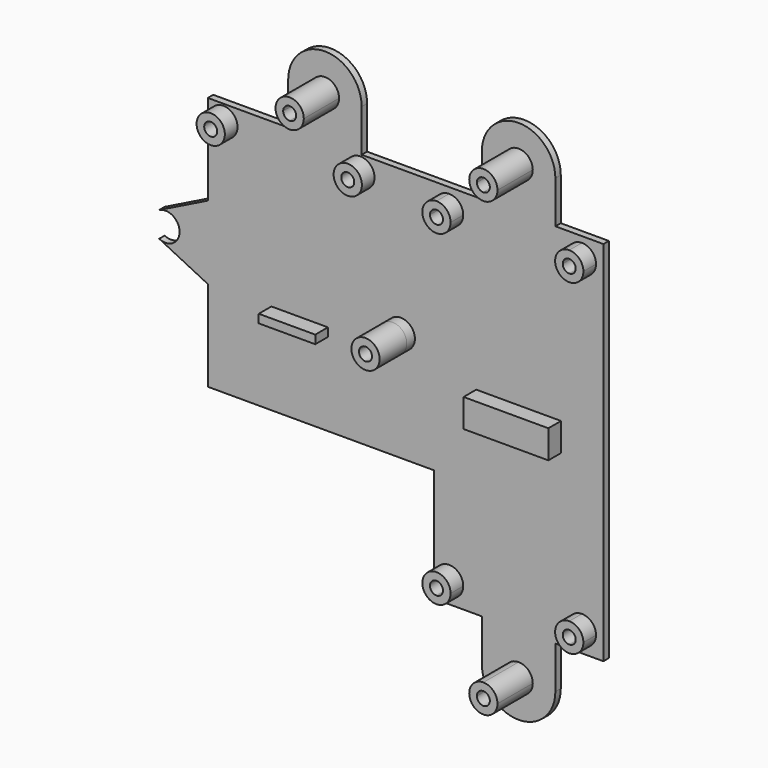
from build123d import *

# Parameters (mm, degrees)
F1_DEPTH = 4
F0_R     = 2.5
F2_DEPTH = 1.2
F3_DEPTH = 9
F0_R_2   = 1.15
F4_DEPTH = 3


# Not quite as in the source:
# - a feature names something its author has since deleted; it is built from what else it names


with BuildPart() as f1:
    # F0 (on Front) → F1 (new body)
    with BuildSketch(Plane.XZ):
        with BuildLine():
            ThreePointArc((-51.5757481032, 29.6725835079), (-54.0757481032, 32.1725835079), (-56.5757481032, 29.6725835079))
            ThreePointArc((-56.5757481032, 29.6725835079), (-54.0757481032, 27.1725835079), (-51.5757481032, 29.6725835079))
        make_face()
        with BuildLine():
            ThreePointArc((-52.9257481032, 29.6725835079), (-54.0757481032, 28.5225835079), (-55.2257481032, 29.6725835079))
            ThreePointArc((-55.2257481032, 29.6725835079), (-54.0757481032, 30.8225835079), (-52.9257481032, 29.6725835079))
        make_face(mode=Mode.SUBTRACT)
    extrude(amount=F1_DEPTH)


with BuildPart() as f1b:
    # F0 (on Front) → F1, piece 2 (new body)
    with BuildSketch(Plane.XZ):
        with BuildLine():
            Line((-28.6757481032, 29.6725835079), (-27.3257481032, 29.6725835079))
            ThreePointArc((-27.3257481032, 29.6725835079), (-29.8257481032, 32.1725835079), (-32.3257481032, 29.6725835079))
            Line((-32.3257481032, 29.6725835079), (-30.9757481032, 29.6725835079))
            ThreePointArc((-30.9757481032, 29.6725835079), (-29.8257481032, 30.8225835079), (-28.6757481032, 29.6725835079))
        make_face()
        with BuildLine():
            ThreePointArc((-32.3257481032, 29.6725835079), (-29.8257481032, 27.1725835079), (-27.3257481032, 29.6725835079))
            Line((-27.3257481032, 29.6725835079), (-28.6757481032, 29.6725835079))
            ThreePointArc((-28.6757481032, 29.6725835079), (-29.8257481032, 28.5225835079), (-30.9757481032, 29.6725835079))
            Line((-30.9757481032, 29.6725835079), (-32.3257481032, 29.6725835079))
        make_face()
    extrude(amount=F1_DEPTH)


with BuildPart() as f1c:
    # F0 (on Front) → F1, piece 3 (new body)
    with BuildSketch(Plane.XZ):
        with BuildLine():
            ThreePointArc((-11.6263987731, 28.95), (-12.3586318202, 30.717766953), (-14.1263987731, 31.45))
            Line((-14.1263987731, 31.45), (-14.1263987731, 30.1))
            ThreePointArc((-14.1263987731, 30.1), (-13.3132259748, 29.7631727984), (-12.9763987731, 28.95))
            Line((-12.9763987731, 28.95), (-11.6263987731, 28.95))
        make_face()
        with BuildLine():
            Line((-14.1263987731, 30.1), (-14.1263987731, 31.45))
            ThreePointArc((-14.1263987731, 31.45), (-15.8941657261, 30.717766953), (-16.6263987731, 28.95))
            Line((-16.6263987731, 28.95), (-15.2763987731, 28.95))
            ThreePointArc((-15.2763987731, 28.95), (-14.9395715715, 29.7631727984), (-14.1263987731, 30.1))
        make_face()
        with BuildLine():
            Line((-15.2763987731, 28.95), (-16.6263987731, 28.95))
            ThreePointArc((-16.6263987731, 28.95), (-16.4189081118, 27.9528034637), (-15.8308780274, 27.1211341023))
            ThreePointArc((-15.8308780274, 27.1211341023), (-13.1292022368, 26.6574906613), (-11.6263987731, 28.95))
            Line((-11.6263987731, 28.95), (-12.9763987731, 28.95))
            ThreePointArc((-12.9763987731, 28.95), (-14.1263987731, 27.8), (-15.2763987731, 28.95))
        make_face()
    extrude(amount=F1_DEPTH)


with BuildPart() as f1d:
    # F0 (on Front) → F1, piece 4 (new body)
    with BuildSketch(Plane.XZ):
        with BuildLine():
            ThreePointArc((9.3736012269, 31.45), (7.6058342739, 30.717766953), (6.8736012269, 28.95))
            Line((6.8736012269, 28.95), (8.2236012269, 28.95))
            ThreePointArc((8.2236012269, 28.95), (8.5604284285, 29.7631727984), (9.3736012269, 30.1))
            Line((9.3736012269, 30.1), (9.3736012269, 31.45))
        make_face()
        with BuildLine():
            Line((8.2236012269, 28.95), (6.8736012269, 28.95))
            ThreePointArc((6.8736012269, 28.95), (7.6058342739, 27.182233047), (9.3736012269, 26.45))
            Line((9.3736012269, 26.45), (9.3736012269, 27.8))
            ThreePointArc((9.3736012269, 27.8), (8.5604284285, 28.1368272016), (8.2236012269, 28.95))
        make_face()
        with BuildLine():
            ThreePointArc((11.8736012269, 28.95), (11.1413681798, 30.717766953), (9.3736012269, 31.45))
            Line((9.3736012269, 31.45), (9.3736012269, 30.1))
            ThreePointArc((9.3736012269, 30.1), (10.1867740252, 29.7631727984), (10.5236012269, 28.95))
            ThreePointArc((10.5236012269, 28.95), (10.1867740252, 28.1368272016), (9.3736012269, 27.8))
            Line((9.3736012269, 27.8), (9.3736012269, 26.45))
            ThreePointArc((9.3736012269, 26.45), (11.1413681798, 27.182233047), (11.8736012269, 28.95))
        make_face()
    extrude(amount=F1_DEPTH)


with BuildPart() as f1e:
    # F0 (on Front) → F1, piece 5 (new body)
    with BuildSketch(Plane.XZ):
        with BuildLine():
            ThreePointArc((-11.6263987731, -28.85), (-15.8941657261, -27.082233047), (-14.1263987731, -31.35))
            ThreePointArc((-14.1263987731, -31.35), (-12.3586318202, -30.617766953), (-11.6263987731, -28.85))
        make_face()
        with BuildLine():
            ThreePointArc((-12.9763987731, -28.85), (-13.3132259748, -29.6631727984), (-14.1263987731, -30))
            ThreePointArc((-14.1263987731, -30), (-14.9395715715, -28.0368272016), (-12.9763987731, -28.85))
        make_face(mode=Mode.SUBTRACT)
    extrude(amount=F1_DEPTH)


with BuildPart() as f1f:
    # F0 (on Front) → F1, piece 6 (new body)
    with BuildSketch(Plane.XZ):
        with BuildLine():
            ThreePointArc((11.8736012269, -28.85), (11.1413681798, -27.082233047), (9.3736012269, -26.35))
            ThreePointArc((9.3736012269, -26.35), (6.8736012269, -28.85), (9.3736012269, -31.35))
            ThreePointArc((9.3736012269, -31.35), (11.1413681798, -30.617766953), (11.8736012269, -28.85))
        make_face()
        with BuildLine():
            ThreePointArc((10.5236012269, -28.85), (10.1867740252, -29.6631727984), (9.3736012269, -30))
            ThreePointArc((9.3736012269, -30), (8.5604284285, -28.0368272016), (10.5236012269, -28.85))
        make_face(mode=Mode.SUBTRACT)
    extrude(amount=F1_DEPTH)


with BuildPart() as f1g:
    # F0 (on Front) → F1, piece 7 (new body)
    with BuildSketch(Plane.XZ):
        Polygon((-35.5757481032, 3.6725835079), (-40.5757481032, 3.6725835079), (-45.5757481032, 3.6725835079), (-45.5757481032, 2.1725835079), (-35.5757481032, 2.1725835079), align=None)
    extrude(amount=F1_DEPTH)


with BuildPart() as f1h:
    # F0 (on Front) → F1, piece 8 (new body)
    with BuildSketch(Plane.XZ):
        Polygon((5.6736012269, 2.5), (-1.8263987731, 2.5), (-9.3263987731, 2.5), (-9.3263987731, -2.5), (5.6736012269, -2.5), align=None)
    extrude(amount=F1_DEPTH)


with BuildPart() as f2:
    # F0 (on Front) → F2 (new body)
    with BuildSketch(Plane.XZ):
        with BuildLine():
            Line((-14.1263987731, 32.5), (-16.8263987731, 32.5))
            Line((-16.8263987731, 32.5), (-16.8263987731, 28.95))
            Line((-16.8263987731, 28.95), (-16.6263987731, 28.95))
            ThreePointArc((-16.6263987731, 28.95), (-15.8941657261, 30.717766953), (-14.1263987731, 31.45))
            Line((-14.1263987731, 31.45), (-14.1263987731, 32.5))
        make_face()
        with BuildLine():
            Line((-16.8263987731, 28.95), (-16.8263987731, 32.5))
            Line((-16.8263987731, 32.5), (-29.6046157777, 32.5))
            Line((-29.6046157777, 32.5), (-36.1046157777, 32.5))
            Line((-36.1046157777, 32.5), (-42.6046157777, 32.5))
            Line((-42.6046157777, 32.5), (-56.8263987731, 32.5))
            Line((-56.8263987731, 32.5), (-56.8263987731, 29.6725835079))
            Line((-56.8263987731, 29.6725835079), (-56.5757481032, 29.6725835079))
            ThreePointArc((-56.5757481032, 29.6725835079), (-54.0757481032, 32.1725835079), (-51.5757481032, 29.6725835079))
            Line((-51.5757481032, 29.6725835079), (-51.3257481032, 29.6725835079))
            Line((-51.3257481032, 29.6725835079), (-40.5757481032, 29.6725835079))
            Line((-40.5757481032, 29.6725835079), (-32.3257481032, 29.6725835079))
            ThreePointArc((-32.3257481032, 29.6725835079), (-29.8257481032, 32.1725835079), (-27.3257481032, 29.6725835079))
            Line((-27.3257481032, 29.6725835079), (-27.3257481032, 20.5483327715))
            Line((-27.3257481032, 20.5483327715), (-16.8263987731, 20.68381793))
            Line((-16.8263987731, 20.68381793), (-16.8263987731, 27.1211341023))
            Line((-16.8263987731, 27.1211341023), (-16.8263987731, 28.95))
        make_face()
        with BuildLine():
            Line((-8.3263987731, 32.5), (-14.1263987731, 32.5))
            Line((-14.1263987731, 32.5), (-14.1263987731, 31.45))
            ThreePointArc((-14.1263987731, 31.45), (-12.3586318202, 30.717766953), (-11.6263987731, 28.95))
            Line((-11.6263987731, 28.95), (-1.8263987731, 28.95))
            Line((-1.8263987731, 28.95), (-1.8263987731, 32.5))
            Line((-1.8263987731, 32.5), (-8.3263987731, 32.5))
        make_face()
        with BuildLine():
            Line((-16.6263987731, 28.95), (-16.8263987731, 28.95))
            Line((-16.8263987731, 28.95), (-16.8263987731, 27.1211341023))
            Line((-16.8263987731, 27.1211341023), (-15.8308780274, 27.1211341023))
            ThreePointArc((-15.8308780274, 27.1211341023), (-16.4189081118, 27.9528034637), (-16.6263987731, 28.95))
        make_face()
        with BuildLine():
            Line((-36.1046157777, 32.5), (-29.6046157777, 32.5))
            Line((-29.6046157777, 32.5), (-29.6046157777, 40))
            ThreePointArc((-29.6046157777, 40), (-31.5084217, 35.4038059223), (-36.1046157777, 33.5))
            Line((-36.1046157777, 33.5), (-36.1046157777, 32.5))
        make_face()
        with BuildLine():
            Line((-8.3263987731, 40), (-8.3263987731, 32.5))
            Line((-8.3263987731, 32.5), (-1.8263987731, 32.5))
            Line((-1.8263987731, 32.5), (-1.8263987731, 33.5))
            ThreePointArc((-1.8263987731, 33.5), (-6.4225928508, 35.4038059223), (-8.3263987731, 40))
        make_face()
        with BuildLine():
            Line((-15.8308780274, 27.1211341023), (-16.8263987731, 27.1211341023))
            Line((-16.8263987731, 27.1211341023), (-16.8263987731, 20.68381793))
            Line((-16.8263987731, 20.68381793), (-16.8263987731, 10))
            Line((-16.8263987731, 10), (-1.8263987731, 10))
            Line((-1.8263987731, 10), (-1.8263987731, 28.95))
            Line((-1.8263987731, 28.95), (-11.6263987731, 28.95))
            ThreePointArc((-11.6263987731, 28.95), (-13.1292022368, 26.6574906613), (-15.8308780274, 27.1211341023))
        make_face()
        with BuildLine():
            Line((-42.6046157777, 32.5), (-36.1046157777, 32.5))
            Line((-36.1046157777, 32.5), (-36.1046157777, 33.5))
            ThreePointArc((-36.1046157777, 33.5), (-40.7008098554, 35.4038059223), (-42.6046157777, 40))
            Line((-42.6046157777, 40), (-42.6046157777, 32.5))
        make_face()
        with BuildLine():
            Line((-33.6046157777, 40), (-29.6046157777, 40))
            ThreePointArc((-29.6046157777, 40), (-36.1046157777, 46.5), (-42.6046157777, 40))
            Line((-42.6046157777, 40), (-38.6046157777, 40))
            ThreePointArc((-38.6046157777, 40), (-36.1046157777, 42.5), (-33.6046157777, 40))
        make_face()
        with BuildLine():
            ThreePointArc((-36.1046157777, 33.5), (-31.5084217, 35.4038059223), (-29.6046157777, 40))
            Line((-29.6046157777, 40), (-33.6046157777, 40))
            ThreePointArc((-33.6046157777, 40), (-34.3368488248, 38.232233047), (-36.1046157777, 37.5))
            Line((-36.1046157777, 37.5), (-36.1046157777, 33.5))
        make_face()
        with BuildLine():
            Line((-1.8263987731, 33.5), (-1.8263987731, 32.5))
            Line((-1.8263987731, 32.5), (4.6736012269, 32.5))
            Line((4.6736012269, 32.5), (4.6736012269, 40))
            ThreePointArc((4.6736012269, 40), (2.7697953046, 35.4038059223), (-1.8263987731, 33.5))
        make_face()
        with BuildLine():
            Line((4.6736012269, 32.5), (-1.8263987731, 32.5))
            Line((-1.8263987731, 32.5), (-1.8263987731, 28.95))
            Line((-1.8263987731, 28.95), (6.8736012269, 28.95))
            ThreePointArc((6.8736012269, 28.95), (7.6058342739, 30.717766953), (9.3736012269, 31.45))
            Line((9.3736012269, 31.45), (9.3736012269, 32.5))
            Line((9.3736012269, 32.5), (4.6736012269, 32.5))
        make_face()
        with BuildLine():
            Line((-4.3263987731, 40), (-8.3263987731, 40))
            ThreePointArc((-8.3263987731, 40), (-6.4225928508, 35.4038059223), (-1.8263987731, 33.5))
            Line((-1.8263987731, 33.5), (-1.8263987731, 37.5))
            ThreePointArc((-1.8263987731, 37.5), (-3.5941657261, 38.232233047), (-4.3263987731, 40))
        make_face()
        with BuildLine():
            ThreePointArc((4.6736012269, 40), (-1.8263987731, 46.5), (-8.3263987731, 40))
            Line((-8.3263987731, 40), (-4.3263987731, 40))
            ThreePointArc((-4.3263987731, 40), (-1.8263987731, 42.5), (0.6736012269, 40))
            Line((0.6736012269, 40), (4.6736012269, 40))
        make_face()
        Polygon((-16.8263987731, 10), (-16.8263987731, 20.68381793), (-27.3257481032, 20.5483327715), (-27.3257481032, 10), align=None)
        with BuildLine():
            ThreePointArc((-42.6046157777, 40), (-40.7008098554, 35.4038059223), (-36.1046157777, 33.5))
            Line((-36.1046157777, 33.5), (-36.1046157777, 37.5))
            ThreePointArc((-36.1046157777, 37.5), (-37.8723827307, 38.232233047), (-38.6046157777, 40))
            Line((-38.6046157777, 40), (-42.6046157777, 40))
        make_face()
        with BuildLine():
            Line((6.8736012269, 28.95), (-1.8263987731, 28.95))
            Line((-1.8263987731, 28.95), (-1.8263987731, 10))
            Line((-1.8263987731, 10), (9.3736012269, 10))
            Line((9.3736012269, 10), (9.3736012269, 26.45))
            ThreePointArc((9.3736012269, 26.45), (7.6058342739, 27.182233047), (6.8736012269, 28.95))
        make_face()
        with BuildLine():
            Line((-1.8263987731, 37.5), (-1.8263987731, 33.5))
            ThreePointArc((-1.8263987731, 33.5), (2.7697953046, 35.4038059223), (4.6736012269, 40))
            Line((4.6736012269, 40), (0.6736012269, 40))
            ThreePointArc((0.6736012269, 40), (-0.0586318202, 38.232233047), (-1.8263987731, 37.5))
        make_face()
        with BuildLine():
            Line((-1.8263987731, 10), (-16.8263987731, 10))
            Line((-16.8263987731, 10), (-16.8263987731, -12.5))
            Line((-16.8263987731, -12.5), (-16.8263987731, -32.5))
            Line((-16.8263987731, -32.5), (-14.1263987731, -32.5))
            Line((-14.1263987731, -32.5), (-8.3263987731, -32.5))
            Line((-8.3263987731, -32.5), (-1.8263987731, -32.5))
            Line((-1.8263987731, -32.5), (4.6736012269, -32.5))
            Line((4.6736012269, -32.5), (9.3736012269, -32.5))
            Line((9.3736012269, -32.5), (9.3736012269, -31.35))
            ThreePointArc((9.3736012269, -31.35), (6.8736012269, -28.85), (9.3736012269, -26.35))
            Line((9.3736012269, -26.35), (9.3736012269, 10))
            Line((9.3736012269, 10), (-1.8263987731, 10))
        make_face()
        with BuildLine():
            ThreePointArc((-11.6263987731, -28.85), (-12.3586318202, -30.617766953), (-14.1263987731, -31.35))
            ThreePointArc((-14.1263987731, -31.35), (-15.8941657261, -27.082233047), (-11.6263987731, -28.85))
        make_face(mode=Mode.SUBTRACT)
        Polygon((-9.3263987731, 2.5), (-1.8263987731, 2.5), (5.6736012269, 2.5), (5.6736012269, -2.5), (-9.3263987731, -2.5), align=None, mode=Mode.SUBTRACT)
        Polygon((-16.8263987731, -12.5), (-16.8263987731, 10), (-27.3257481032, 10), (-40.5757481032, 10), (-56.8263987731, 10), (-56.8263987731, 3.5), (-56.8263987731, -12.5), align=None)
        Polygon((-45.5757481032, 3.6725835079), (-40.5757481032, 3.6725835079), (-35.5757481032, 3.6725835079), (-35.5757481032, 2.1725835079), (-45.5757481032, 2.1725835079), align=None, mode=Mode.SUBTRACT)
        with Locations((-22.6864659105, 6.8783217843)):
            Circle(F0_R, mode=Mode.SUBTRACT)
        with BuildLine():
            Line((-27.3257481032, 10), (-27.3257481032, 20.5483327715))
            Line((-27.3257481032, 20.5483327715), (-27.3257481032, 29.6725835079))
            ThreePointArc((-27.3257481032, 29.6725835079), (-29.8257481032, 27.1725835079), (-32.3257481032, 29.6725835079))
            Line((-32.3257481032, 29.6725835079), (-40.5757481032, 29.6725835079))
            Line((-40.5757481032, 29.6725835079), (-40.5757481032, 10))
            Line((-40.5757481032, 10), (-27.3257481032, 10))
        make_face()
        with BuildLine():
            Line((13.1736012269, 32.5), (9.3736012269, 32.5))
            Line((9.3736012269, 32.5), (9.3736012269, 31.45))
            ThreePointArc((9.3736012269, 31.45), (11.1413681798, 30.717766953), (11.8736012269, 28.95))
            ThreePointArc((11.8736012269, 28.95), (11.1413681798, 27.182233047), (9.3736012269, 26.45))
            Line((9.3736012269, 26.45), (9.3736012269, 10))
            Line((9.3736012269, 10), (13.1736012269, 10))
            Line((13.1736012269, 10), (13.1736012269, 32.5))
        make_face()
        with BuildLine():
            Line((-56.5757481032, 29.6725835079), (-56.8263987731, 29.6725835079))
            Line((-56.8263987731, 29.6725835079), (-56.8263987731, 16.5))
            Line((-56.8263987731, 16.5), (-56.8263987731, 10))
            Line((-56.8263987731, 10), (-40.5757481032, 10))
            Line((-40.5757481032, 10), (-40.5757481032, 29.6725835079))
            Line((-40.5757481032, 29.6725835079), (-51.3257481032, 29.6725835079))
            Line((-51.3257481032, 29.6725835079), (-51.5757481032, 29.6725835079))
            ThreePointArc((-51.5757481032, 29.6725835079), (-54.0757481032, 27.1725835079), (-56.5757481032, 29.6725835079))
        make_face()
        with BuildLine():
            Line((13.1736012269, 10), (9.3736012269, 10))
            Line((9.3736012269, 10), (9.3736012269, -26.35))
            ThreePointArc((9.3736012269, -26.35), (11.1413681798, -27.082233047), (11.8736012269, -28.85))
            ThreePointArc((11.8736012269, -28.85), (11.1413681798, -30.617766953), (9.3736012269, -31.35))
            Line((9.3736012269, -31.35), (9.3736012269, -32.5))
            Line((9.3736012269, -32.5), (13.1736012269, -32.5))
            Line((13.1736012269, -32.5), (13.1736012269, 10))
        make_face()
        with BuildLine():
            Line((-56.8263987731, 10), (-56.8263987731, 16.5))
            Line((-56.8263987731, 16.5), (-65.4350399232, 12.2407397886))
            ThreePointArc((-65.4350399232, 12.2407397886), (-63.0076119964, 12.1238647409), (-61.8263987731, 10))
            Line((-61.8263987731, 10), (-56.8263987731, 10))
        make_face()
        with BuildLine():
            Line((-65.4350399232, 7.7592602114), (-56.8263987731, 3.5))
            Line((-56.8263987731, 3.5), (-56.8263987731, 10))
            Line((-56.8263987731, 10), (-61.8263987731, 10))
            ThreePointArc((-61.8263987731, 10), (-63.0076119964, 7.8761352591), (-65.4350399232, 7.7592602114))
        make_face()
        with BuildLine():
            Line((-1.8263987731, -32.5), (-8.3263987731, -32.5))
            Line((-8.3263987731, -32.5), (-8.3263987731, -40))
            ThreePointArc((-8.3263987731, -40), (-6.4225928508, -35.4038059223), (-1.8263987731, -33.5))
            Line((-1.8263987731, -33.5), (-1.8263987731, -32.5))
        make_face()
        with BuildLine():
            Line((4.6736012269, -32.5), (-1.8263987731, -32.5))
            Line((-1.8263987731, -32.5), (-1.8263987731, -33.5))
            ThreePointArc((-1.8263987731, -33.5), (2.7697953046, -35.4038059223), (4.6736012269, -40))
            Line((4.6736012269, -40), (4.6736012269, -32.5))
        make_face()
        with BuildLine():
            Line((-4.3263987731, -40), (-8.3263987731, -40))
            ThreePointArc((-8.3263987731, -40), (-1.8263987731, -46.5), (4.6736012269, -40))
            Line((4.6736012269, -40), (0.6736012269, -40))
            ThreePointArc((0.6736012269, -40), (-1.8263987731, -42.5), (-4.3263987731, -40))
        make_face()
        with BuildLine():
            ThreePointArc((-1.8263987731, -33.5), (-6.4225928508, -35.4038059223), (-8.3263987731, -40))
            Line((-8.3263987731, -40), (-4.3263987731, -40))
            ThreePointArc((-4.3263987731, -40), (-3.5941657261, -38.232233047), (-1.8263987731, -37.5))
            Line((-1.8263987731, -37.5), (-1.8263987731, -33.5))
        make_face()
        with BuildLine():
            ThreePointArc((4.6736012269, -40), (2.7697953046, -35.4038059223), (-1.8263987731, -33.5))
            Line((-1.8263987731, -33.5), (-1.8263987731, -37.5))
            ThreePointArc((-1.8263987731, -37.5), (-0.0586318202, -38.232233047), (0.6736012269, -40))
            Line((0.6736012269, -40), (4.6736012269, -40))
        make_face()
    extrude(amount=F2_DEPTH)


with BuildPart() as f2b:
    # F0 (on Front) → F2, piece 2 (new body)
    with BuildSketch(Plane.XZ):
        with BuildLine():
            Line((-14.1263987731, 28.95), (-14.1263987731, 30.1))
            ThreePointArc((-14.1263987731, 30.1), (-14.9395715715, 29.7631727984), (-15.2763987731, 28.95))
            Line((-15.2763987731, 28.95), (-14.1263987731, 28.95))
        make_face()
        with BuildLine():
            ThreePointArc((-12.9763987731, 28.95), (-13.3132259748, 29.7631727984), (-14.1263987731, 30.1))
            Line((-14.1263987731, 30.1), (-14.1263987731, 28.95))
            Line((-14.1263987731, 28.95), (-12.9763987731, 28.95))
        make_face()
        with BuildLine():
            Line((-14.1263987731, 28.95), (-15.2763987731, 28.95))
            ThreePointArc((-15.2763987731, 28.95), (-14.1263987731, 27.8), (-12.9763987731, 28.95))
            Line((-12.9763987731, 28.95), (-14.1263987731, 28.95))
        make_face()
    extrude(amount=F2_DEPTH)


with BuildPart() as f2c:
    # F0 (on Front) → F2, piece 3 (new body)
    with BuildSketch(Plane.XZ):
        with BuildLine():
            ThreePointArc((-12.9763987731, -28.85), (-14.9395715715, -28.0368272016), (-14.1263987731, -30))
            ThreePointArc((-14.1263987731, -30), (-13.3132259748, -29.6631727984), (-12.9763987731, -28.85))
        make_face()
    extrude(amount=F2_DEPTH)


with BuildPart() as f2d:
    # F0 (on Front) → F2, piece 4 (new body)
    with BuildSketch(Plane.XZ):
        with BuildLine():
            ThreePointArc((9.3736012269, 30.1), (8.5604284285, 29.7631727984), (8.2236012269, 28.95))
            Line((8.2236012269, 28.95), (9.3736012269, 28.95))
            Line((9.3736012269, 28.95), (9.3736012269, 30.1))
        make_face()
        with BuildLine():
            Line((9.3736012269, 28.95), (8.2236012269, 28.95))
            ThreePointArc((8.2236012269, 28.95), (8.5604284285, 28.1368272016), (9.3736012269, 27.8))
            Line((9.3736012269, 27.8), (9.3736012269, 28.95))
        make_face()
        with BuildLine():
            ThreePointArc((10.5236012269, 28.95), (10.1867740252, 29.7631727984), (9.3736012269, 30.1))
            Line((9.3736012269, 30.1), (9.3736012269, 28.95))
            Line((9.3736012269, 28.95), (9.3736012269, 27.8))
            ThreePointArc((9.3736012269, 27.8), (10.1867740252, 28.1368272016), (10.5236012269, 28.95))
        make_face()
    extrude(amount=F2_DEPTH)


with BuildPart() as f2e:
    # F0 (on Front) → F2, piece 5 (new body)
    with BuildSketch(Plane.XZ):
        with BuildLine():
            Line((-29.8257481032, 29.6725835079), (-28.6757481032, 29.6725835079))
            ThreePointArc((-28.6757481032, 29.6725835079), (-29.8257481032, 30.8225835079), (-30.9757481032, 29.6725835079))
            Line((-30.9757481032, 29.6725835079), (-29.8257481032, 29.6725835079))
        make_face()
        with BuildLine():
            ThreePointArc((-30.9757481032, 29.6725835079), (-29.8257481032, 28.5225835079), (-28.6757481032, 29.6725835079))
            Line((-28.6757481032, 29.6725835079), (-29.8257481032, 29.6725835079))
            Line((-29.8257481032, 29.6725835079), (-30.9757481032, 29.6725835079))
        make_face()
    extrude(amount=F2_DEPTH)


with BuildPart() as f2f:
    # F0 (on Front) → F2, piece 6 (new body)
    with BuildSketch(Plane.XZ):
        with BuildLine():
            ThreePointArc((-52.9257481032, 29.6725835079), (-54.0757481032, 30.8225835079), (-55.2257481032, 29.6725835079))
            ThreePointArc((-55.2257481032, 29.6725835079), (-54.0757481032, 28.5225835079), (-52.9257481032, 29.6725835079))
        make_face()
    extrude(amount=F2_DEPTH)


with BuildPart() as f2g:
    # F0 (on Front) → F2, piece 7 (new body)
    with BuildSketch(Plane.XZ):
        with BuildLine():
            ThreePointArc((10.5236012269, -28.85), (8.5604284285, -28.0368272016), (9.3736012269, -30))
            ThreePointArc((9.3736012269, -30), (10.1867740252, -29.6631727984), (10.5236012269, -28.85))
        make_face()
    extrude(amount=F2_DEPTH)


with BuildPart() as f3:
    # F0 (on Front) → F3 (new body)
    with BuildSketch(Plane.XZ):
        with BuildLine():
            Line((-34.9546157777, 40), (-33.6046157777, 40))
            ThreePointArc((-33.6046157777, 40), (-36.1046157777, 42.5), (-38.6046157777, 40))
            Line((-38.6046157777, 40), (-37.2546157777, 40))
            ThreePointArc((-37.2546157777, 40), (-36.1046157777, 41.15), (-34.9546157777, 40))
        make_face()
        with BuildLine():
            ThreePointArc((-36.1046157777, 37.5), (-34.3368488248, 38.232233047), (-33.6046157777, 40))
            Line((-33.6046157777, 40), (-34.9546157777, 40))
            ThreePointArc((-34.9546157777, 40), (-35.2914429794, 39.1868272016), (-36.1046157777, 38.85))
            Line((-36.1046157777, 38.85), (-36.1046157777, 37.5))
        make_face()
        with BuildLine():
            ThreePointArc((-38.6046157777, 40), (-37.8723827307, 38.232233047), (-36.1046157777, 37.5))
            Line((-36.1046157777, 37.5), (-36.1046157777, 38.85))
            ThreePointArc((-36.1046157777, 38.85), (-36.9177885761, 39.1868272016), (-37.2546157777, 40))
            Line((-37.2546157777, 40), (-38.6046157777, 40))
        make_face()
    extrude(amount=F3_DEPTH)


with BuildPart() as f3b:
    # F0 (on Front) → F3, piece 2 (new body)
    with BuildSketch(Plane.XZ):
        with BuildLine():
            Line((-2.9763987731, 40), (-4.3263987731, 40))
            ThreePointArc((-4.3263987731, 40), (-3.5941657261, 38.232233047), (-1.8263987731, 37.5))
            Line((-1.8263987731, 37.5), (-1.8263987731, 38.85))
            ThreePointArc((-1.8263987731, 38.85), (-2.6395715715, 39.1868272016), (-2.9763987731, 40))
        make_face()
        with BuildLine():
            ThreePointArc((0.6736012269, 40), (-1.8263987731, 42.5), (-4.3263987731, 40))
            Line((-4.3263987731, 40), (-2.9763987731, 40))
            ThreePointArc((-2.9763987731, 40), (-1.8263987731, 41.15), (-0.6763987731, 40))
            Line((-0.6763987731, 40), (0.6736012269, 40))
        make_face()
        with BuildLine():
            Line((-1.8263987731, 38.85), (-1.8263987731, 37.5))
            ThreePointArc((-1.8263987731, 37.5), (-0.0586318202, 38.232233047), (0.6736012269, 40))
            Line((0.6736012269, 40), (-0.6763987731, 40))
            ThreePointArc((-0.6763987731, 40), (-1.0132259748, 39.1868272016), (-1.8263987731, 38.85))
        make_face()
    extrude(amount=F3_DEPTH)


with BuildPart() as f3c:
    # F0 (on Front) → F3, piece 3 (new body)
    with BuildSketch(Plane.XZ):
        with BuildLine():
            Line((-2.9763987731, -40), (-4.3263987731, -40))
            ThreePointArc((-4.3263987731, -40), (-1.8263987731, -42.5), (0.6736012269, -40))
            Line((0.6736012269, -40), (-0.6763987731, -40))
            ThreePointArc((-0.6763987731, -40), (-1.8263987731, -41.15), (-2.9763987731, -40))
        make_face()
        with BuildLine():
            ThreePointArc((-1.8263987731, -37.5), (-3.5941657261, -38.232233047), (-4.3263987731, -40))
            Line((-4.3263987731, -40), (-2.9763987731, -40))
            ThreePointArc((-2.9763987731, -40), (-2.6395715715, -39.1868272016), (-1.8263987731, -38.85))
            Line((-1.8263987731, -38.85), (-1.8263987731, -37.5))
        make_face()
        with BuildLine():
            ThreePointArc((0.6736012269, -40), (-0.0586318202, -38.232233047), (-1.8263987731, -37.5))
            Line((-1.8263987731, -37.5), (-1.8263987731, -38.85))
            ThreePointArc((-1.8263987731, -38.85), (-1.0132259748, -39.1868272016), (-0.6763987731, -40))
            Line((-0.6763987731, -40), (0.6736012269, -40))
        make_face()
    extrude(amount=F3_DEPTH)


with BuildPart() as f3d:
    # F0 (on Front) → F3, piece 4 (new body)
    with BuildSketch(Plane.XZ):
        with Locations((-22.6864659105, 6.8783217843)):
            Circle(F0_R)
        with Locations((-22.6864659105, 6.8783217843)):
            Circle(F0_R_2, mode=Mode.SUBTRACT)
    extrude(amount=F3_DEPTH)


with BuildPart() as f4:
    # F0 (on Front) → F4 (new body)
    with BuildSketch(Plane.XZ):
        with BuildLine():
            Line((-1.8263987731, 40), (-2.9763987731, 40))
            ThreePointArc((-2.9763987731, 40), (-2.6395715715, 39.1868272016), (-1.8263987731, 38.85))
            Line((-1.8263987731, 38.85), (-1.8263987731, 40))
        make_face()
        with BuildLine():
            Line((-1.8263987731, 40), (-1.8263987731, 38.85))
            ThreePointArc((-1.8263987731, 38.85), (-1.0132259748, 39.1868272016), (-0.6763987731, 40))
            Line((-0.6763987731, 40), (-1.8263987731, 40))
        make_face()
        with BuildLine():
            ThreePointArc((-0.6763987731, 40), (-1.8263987731, 41.15), (-2.9763987731, 40))
            Line((-2.9763987731, 40), (-1.8263987731, 40))
            Line((-1.8263987731, 40), (-0.6763987731, 40))
        make_face()
    extrude(amount=F4_DEPTH)


with BuildPart() as f4b:
    # F0 (on Front) → F4, piece 2 (new body)
    with BuildSketch(Plane.XZ):
        with BuildLine():
            Line((-36.1046157777, 40), (-34.9546157777, 40))
            ThreePointArc((-34.9546157777, 40), (-36.1046157777, 41.15), (-37.2546157777, 40))
            Line((-37.2546157777, 40), (-36.1046157777, 40))
        make_face()
        with BuildLine():
            ThreePointArc((-36.1046157777, 38.85), (-35.2914429794, 39.1868272016), (-34.9546157777, 40))
            Line((-34.9546157777, 40), (-36.1046157777, 40))
            Line((-36.1046157777, 40), (-36.1046157777, 38.85))
        make_face()
        with BuildLine():
            ThreePointArc((-37.2546157777, 40), (-36.9177885761, 39.1868272016), (-36.1046157777, 38.85))
            Line((-36.1046157777, 38.85), (-36.1046157777, 40))
            Line((-36.1046157777, 40), (-37.2546157777, 40))
        make_face()
    extrude(amount=F4_DEPTH)


with BuildPart() as f4c:
    # F0 (on Front) → F4, piece 3 (new body)
    with BuildSketch(Plane.XZ):
        with BuildLine():
            Line((-1.8263987731, -40), (-2.9763987731, -40))
            ThreePointArc((-2.9763987731, -40), (-1.8263987731, -41.15), (-0.6763987731, -40))
            Line((-0.6763987731, -40), (-1.8263987731, -40))
        make_face()
        with BuildLine():
            ThreePointArc((-1.8263987731, -38.85), (-2.6395715715, -39.1868272016), (-2.9763987731, -40))
            Line((-2.9763987731, -40), (-1.8263987731, -40))
            Line((-1.8263987731, -40), (-1.8263987731, -38.85))
        make_face()
        with BuildLine():
            ThreePointArc((-0.6763987731, -40), (-1.0132259748, -39.1868272016), (-1.8263987731, -38.85))
            Line((-1.8263987731, -38.85), (-1.8263987731, -40))
            Line((-1.8263987731, -40), (-0.6763987731, -40))
        make_face()
    extrude(amount=F4_DEPTH)


with BuildPart() as f4d:
    # F0 (on Front) → F4, piece 4 (new body)
    with BuildSketch(Plane.XZ):
        with Locations((-22.6864659105, 6.8783217843)):
            Circle(F0_R)
        with Locations((-22.6864659105, 6.8783217843)):
            Circle(F0_R_2, mode=Mode.SUBTRACT)
        with Locations((-22.6864659105, 6.8783217843)):
            Circle(F0_R_2)
    extrude(amount=F4_DEPTH)


solid = Compound([f1.part, f1b.part, f1c.part, f1d.part, f1e.part, f1f.part, f1g.part, f1h.part, f2.part, f2b.part, f2c.part, f2d.part, f2e.part, f2f.part, f2g.part, f3.part, f3b.part, f3c.part, f3d.part, f4.part, f4b.part, f4c.part, f4d.part])
